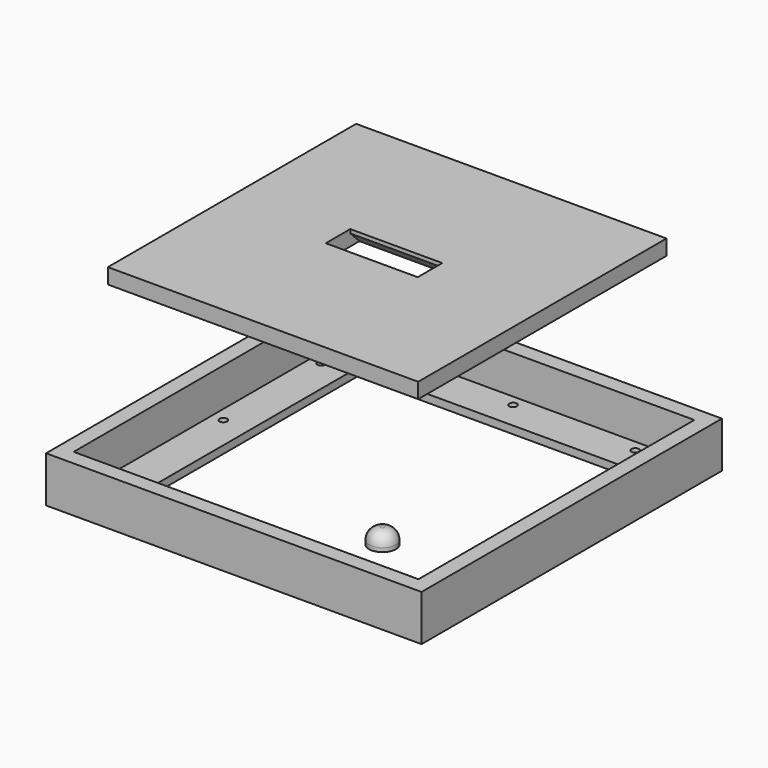
from build123d import *

# Parameters (mm, degrees)
F0_W      = 49
F0_H      = 49
F1_DEPTH  = 6
F2_W      = 45
F2_H      = 45
F3_DEPTH  = 5
F4_W      = 35
F4_H      = 35
F5_DEPTH  = 6.001
F10_W     = 40.5
F10_H     = 40.5
F11_DEPTH = 2
F12_W     = 12
F12_H     = 4
F13_DEPTH = 33.3483119268
F14_SIZE  = 1.5
F15_R     = 0.5
F16_DEPTH = 1


# Not quite as in the source:
# - a feature of the source that left no trace in its solid (it failed there, or was rolled back) is left out


with BuildPart() as f1:
    # F0 (on Top) → F1 (new body)
    with BuildSketch(Plane.XY):
        Rectangle(F0_W, F0_H)
    extrude(amount=F1_DEPTH)

    # F2 (on face) → F3 (cut)
    with BuildSketch(Plane.XY.offset(6)):
        Rectangle(F2_W, F2_H)
    extrude(amount=-F3_DEPTH, mode=Mode.SUBTRACT)

    # F4 (on face) → F5 (cut, through all)
    with BuildSketch(Plane(origin=(0, 0, 0), x_dir=(1, 0, 0), z_dir=(0, 0, -1))):
        Rectangle(F4_W, F4_H)
    extrude(amount=-F5_DEPTH, mode=Mode.SUBTRACT)

    # F15 (on face) → F16 (cut)
    with BuildSketch(Plane(origin=(0, 0, 0), x_dir=(1, 0, 0), z_dir=(0, 0, -1))):
        with Locations((0, 20.8953134716)):
            Circle(F15_R)
        with Locations((-20.9677405655, 0)):
            Circle(F15_R)
        with Locations((0, -21.0554059595)):
            Circle(F15_R)
        with Locations((21.0171975195, 0)):
            Circle(F15_R)
        with Locations((21, 16.0074820742)):
            Circle(F15_R)
        with Locations((15.9945003688, 20.9227129817)):
            Circle(F15_R)
        with Locations((-16.0156711936, 21)):
            Circle(F15_R)
        with Locations((-21, 16.0026811063)):
            Circle(F15_R)
        with Locations((-21, -15.9993395209)):
            Circle(F15_R)
        with Locations((-16.001984477, -21)):
            Circle(F15_R)
        with Locations((15.9951094538, -21)):
            Circle(F15_R)
        with Locations((21, -16.0031374544)):
            Circle(F15_R)
    extrude(amount=-F16_DEPTH, mode=Mode.SUBTRACT)


with BuildPart() as f8:
    # F7 (on Right) → F8 (revolve)
    with BuildSketch(Plane.YZ):
        with BuildLine():
            Line((-2.0008900769, -5.8473119268), (-2.0008900769, -6.3473119268))
            Line((-2.0008900769, -6.3473119268), (-0.2508900769, -6.3473119268))
            Line((-0.2508900769, -6.3473119268), (-0.2508900769, -4.3473119268))
            Line((-0.2508900769, -4.3473119268), (-0.5008900769, -4.3473119268))
            ThreePointArc((-0.5008900769, -4.3473119268), (-1.5615502487, -4.786651755), (-2.0008900769, -5.8473119268))
        make_face()
    revolve(axis=Axis((0, -0.2508900769, -5.3473119268), (0, 0, 1)))


with BuildPart() as f11:
    # F10 (on offset) → F11 (new body)
    with BuildSketch(Plane.XY.offset(25)):
        with Locations((0.2051311374, 0.2580289319)):
            Rectangle(F10_W, F10_H)
    extrude(amount=F11_DEPTH)

    # F12 (on face) → F13 (cut, through all)
    with BuildSketch(Plane.XY.offset(27)):
        Rectangle(F12_W, F12_H)
    extrude(amount=-F13_DEPTH, mode=Mode.SUBTRACT)

    # F14
    f14_edges = [f11.edges().sort_by_distance(p)[0] for p in [
        (0, -2, 25),
        (0, 2, 25),
    ]]
    chamfer(f14_edges, length=F14_SIZE)


solid = Compound([f1.part, f8.part, f11.part])
